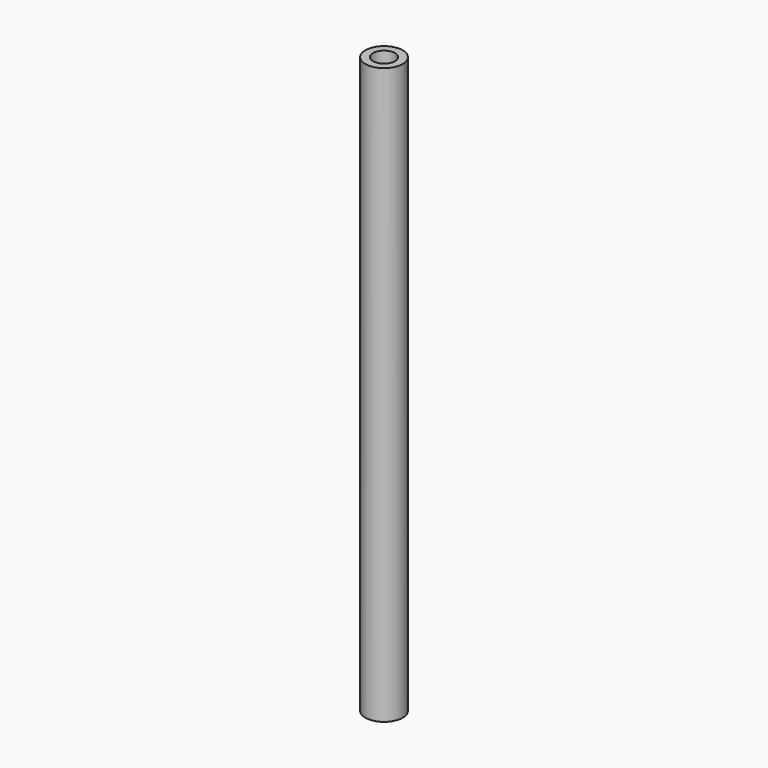
from build123d import *

# Parameters (mm, degrees)
F1_R     = 10.715625
F1_R_2   = 6.35
F2_DEPTH = 330.2


# Not quite as in the source:
# - a variable given as a bare number and used for a length is read in inches; the dataset says mm whatever the document's units were


with BuildPart() as f2:
    # F1 (on Top) → F2 (new body)
    with BuildSketch(Plane.XY):
        Circle(F1_R)
        Circle(F1_R_2, mode=Mode.SUBTRACT)
    extrude(amount=F2_DEPTH)


solid = f2.part
